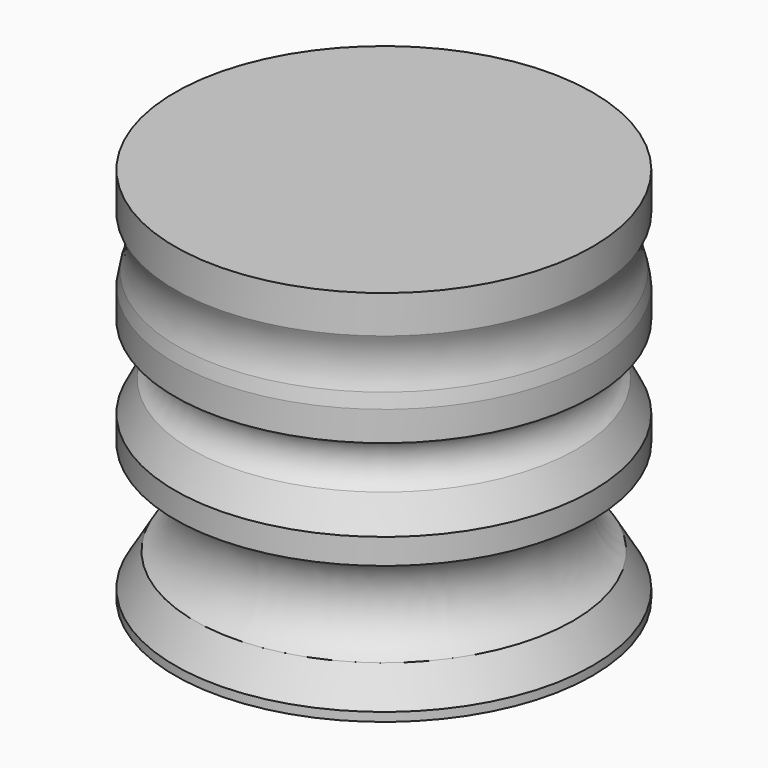
from build123d import *


# Not quite as in the source:
# - a fillet or chamfer that OpenCascade refuses, or shapes differently, is made with other operations: its cross-section is extruded or revolved along the edge and cut away or added


with BuildPart() as f1:
    # F0 (on Front) → F1 (revolve)
    with BuildSketch(Plane.XZ):
        with BuildLine():
            Line((0, 0), (70.2457263553, 0))
            Line((70.2457263553, 0), (70.2457263553, 12.037278153))
            ThreePointArc((70.2457263553, 12.037278153), (54.7893275552, 29.1168470867), (70.2457263553, 46.1964160204))
            Line((70.2457263553, 46.1964160204), (70.2457263553, 63.5))
            ThreePointArc((70.2457263553, 63.5), (60.7207263553, 73.025), (70.2457263553, 82.55))
            Line((70.2457263553, 82.55), (70.2457263553, 95.25))
            ThreePointArc((70.2457263553, 95.25), (67.9381906617, 104.775), (70.2457263553, 114.3))
            Line((70.2457263553, 114.3), (70.2457263553, 127))
            Line((70.2457263553, 127), (0, 127))
            Line((0, 127), (0, 0))
        make_face()
    revolve(axis=Axis((0, 0, 63.5), (0, 0, 1)))

    # F2: chamfer of 12.7 on 3 edges, made by hand

    # F2_s1 → F2_t2 (revolve, cut)
    with BuildSketch(Plane.XZ):
        with BuildLine():
            Line((70.2457263553, 54.7860135972), (64.8028692124, 65.2082915417))
            ThreePointArc((64.8028692124, 65.2082915417), (67.2107952899, 63.9964442778), (70.2457263553, 63.5))
            Line((70.2457263553, 63.5), (70.2457263553, 54.7860135972))
        make_face()
    revolve(axis=Axis((0, 0, 63.5), (0, 0, 1)), mode=Mode.SUBTRACT)

    # F2_s3 → F2_t4 (revolve, cut)
    with BuildSketch(Plane.XZ):
        with BuildLine():
            Line((70.2457263553, 92.5546468293), (69.3712508592, 97.1857341969))
            ThreePointArc((69.3712508592, 97.1857341969), (69.6830735003, 96.4332072381), (70.2457263553, 95.25))
            Line((70.2457263553, 95.25), (70.2457263553, 92.5546468293))
        make_face()
    revolve(axis=Axis((0, 0, 95.25), (0, 0, 1)), mode=Mode.SUBTRACT)

    # F2_s5 → F2_t6 (revolve, cut)
    with BuildSketch(Plane.XZ):
        with BuildLine():
            Line((70.2457263553, 2.9576382974), (63.6728956225, 14.0818369998))
            ThreePointArc((63.6728956225, 14.0818369998), (66.6706692782, 12.7854237046), (70.2457263553, 12.037278153))
            Line((70.2457263553, 12.037278153), (70.2457263553, 2.9576382974))
        make_face()
    revolve(axis=Axis((0, 0, 12.037278153), (0, 0, 1)), mode=Mode.SUBTRACT)


solid = f1.part
